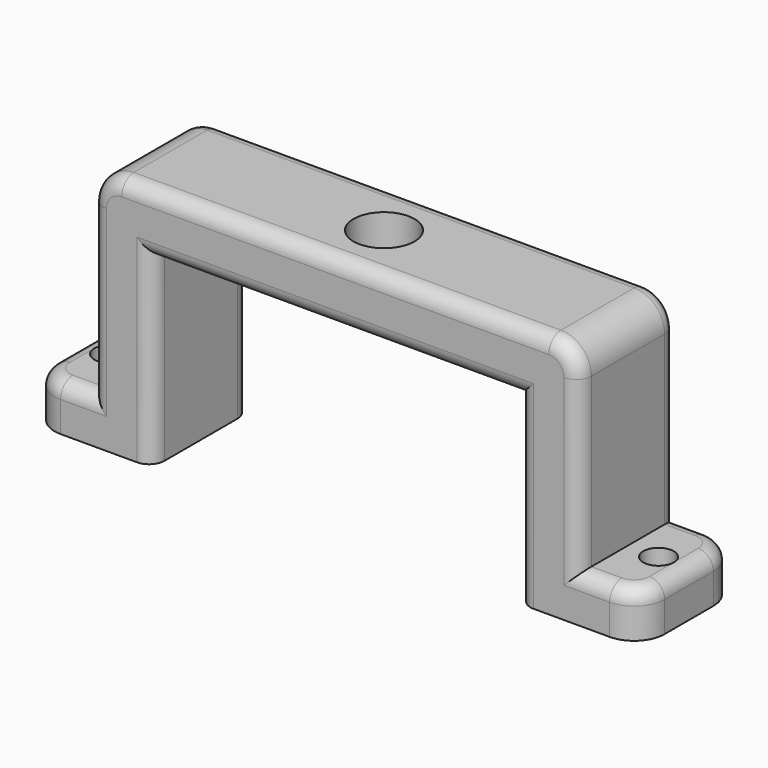
from build123d import *

# Parameters (mm, degrees)
F1_DEPTH = 12.7
F2_R     = 3.175
F3_DEPTH = 9.526
F4_R     = 6.35
F5_DEPTH = 50.801
F6_R     = 6.35
F7_R     = 3.17499


# Not quite as in the source:
# - a fillet or chamfer is up to 0.001 mm smaller than in the source, because OpenCascade refuses the exact size


with BuildPart() as f1:
    # F0 (on Front) → F1 (new body, symmetric)
    with BuildSketch(Plane.XZ):
        Polygon((-50.8, -22.066242151), (-63.5, -22.066242151), (-63.5, -31.591242151), (-38.1, -31.591242151), (-38.1, 6.508757849), (0, 6.508757849), (38.1, 6.508757849), (38.1, -31.591242151), (63.5, -31.591242151), (63.5, -22.066242151), (50.8, -22.066242151), (50.8, 19.208757849), (0, 19.208757849), (-50.8, 19.208757849), align=None)
    extrude(amount=F1_DEPTH, both=True)

    # F2 (on face) → F3 (cut, through all)
    with BuildSketch(Plane.XY.offset(-22.066242151)):
        with Locations((-57.15, 0)):
            Circle(F2_R)
        with Locations((57.15, 0)):
            Circle(F2_R)
    extrude(amount=-F3_DEPTH, mode=Mode.SUBTRACT)

    # F4 (on face) → F5 (cut, through all)
    with BuildSketch(Plane.XY.offset(19.208757849)):
        Circle(F4_R)
    extrude(amount=-F5_DEPTH, mode=Mode.SUBTRACT)

    # F6
    f6_edges = [f1.edges().sort_by_distance(p)[0] for p in [
        (-50.8, 0, 19.208758),
        (50.8, 0, 19.208758),
        (-63.5, -12.7, -26.828742),
        (63.5, -12.7, -26.828742),
        (63.5, 12.7, -26.828742),
        (-63.5, 12.7, -26.828742),
    ]]
    fillet(f6_edges, radius=F6_R)

    # F7 (radius 3.175 in the source; OpenCascade refuses exactly that, so slightly less here)
    f7_edges = [f1.edges().sort_by_distance(p)[0] for p in [
        (-50.8, -12.7, -4.603742),
        (-53.975, -12.7, -22.066242),
        (-38.1, -12.7, -12.541242),
        (0, -12.7, 6.508758),
        (38.1, -12.7, -12.541242),
        (50.8, 12.7, -4.603742),
        (53.975, 12.7, -22.066242),
        (38.1, 12.7, -12.541242),
        (0, 12.7, 6.508758),
        (-38.1, 12.7, -12.541242),
    ]]
    fillet(f7_edges, radius=F7_R)


solid = f1.part
